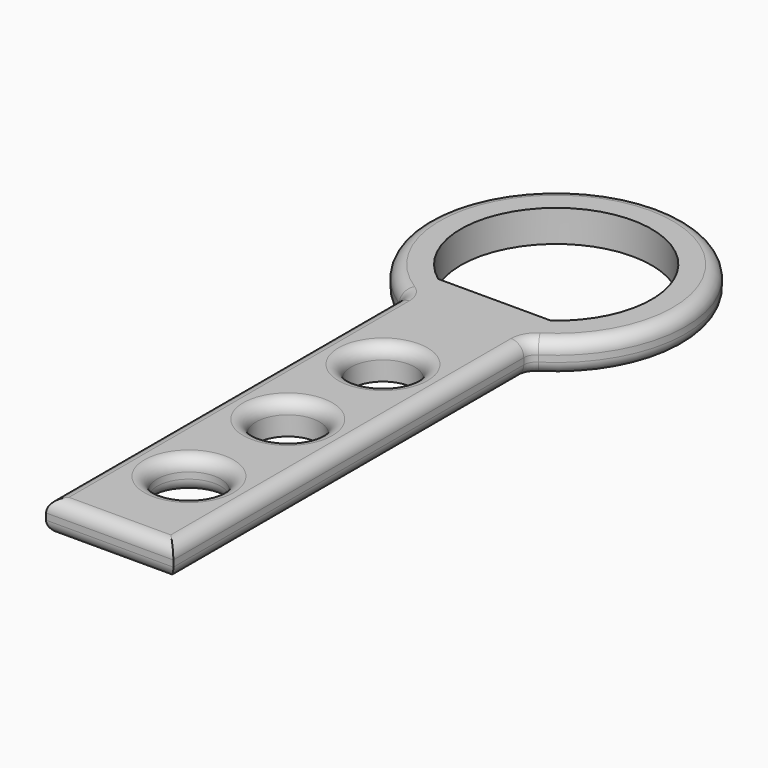
from build123d import *

# Parameters (mm, degrees)
F1_DEPTH = 5
F2_R     = 2
F3_R     = 15
F4_DEPTH = 25.4
F5_R     = 5
F6_DEPTH = 25.4
F7_R     = 2
F9_DEPTH = 5
F10_SIZE = 4.99999


# Not quite as in the source:
# - a fillet or chamfer is up to 0.001 mm smaller than in the source, because OpenCascade refuses the exact size


with BuildPart() as f1:
    # F0 (on Top) → F1 (new body)
    with BuildSketch(Plane.XY):
        with BuildLine():
            Line((-10, -35), (10, -35))
            Line((10, -35), (10, 35))
            ThreePointArc((10, 35), (0, 73.0924170341), (-10, 35))
            Line((-10, 35), (-10, -35))
        make_face()
    extrude(amount=F1_DEPTH)

    # F2
    f2_edges = [f1.edges().sort_by_distance(p)[0] for p in [
        (0, 73.092417, 5),
        (10, 0, 5),
        (-10, 0, 5),
        (0, -35, 5),
        (10, 0, 0),
        (0, 73.092417, 0),
        (-10, 0, 0),
        (-10, 35, 2.5),
        (10, 35, 2.5),
        (0, -35, 0),
    ]]
    fillet(f2_edges, radius=F2_R)

    # F3 (on face) → F4 (cut)
    with BuildSketch(Plane.XY.offset(5)):
        with Locations((0, 52.7336113155)):
            Circle(F3_R)
    extrude(amount=-F4_DEPTH, mode=Mode.SUBTRACT)

    # F5 (on face) → F6 (cut)
    with BuildSketch(Plane(origin=(0, 0, 0), x_dir=(1, 0, 0), z_dir=(0, 0, -1))):
        Circle(F5_R)
        with Locations((0, -18.6964944005)):
            Circle(F5_R)
        with Locations((0, 19.4296911359)):
            Circle(F5_R)
    extrude(amount=-F6_DEPTH, mode=Mode.SUBTRACT)

    # F7
    f7_edges = [f1.edges().sort_by_distance(p)[0] for p in [
        (-5, -19.429691, 0),
        (5, -19.429691, 2.5),
        (-5, -19.429691, 5),
        (-5, 0, 5),
        (-5, 18.696494, 5),
    ]]
    fillet(f7_edges, radius=F7_R)

    # F8 (on face) → F9 (join)
    with BuildSketch(Plane(origin=(0, 0, 0), x_dir=(1, 0, 0), z_dir=(0, 0, -1))):
        with BuildLine():
            ThreePointArc((13.2130736886, -45.6332814852), (0, -37.7336113155), (-13.2130736886, -45.6332814852))
            Line((-13.2130736886, -45.6332814852), (13.2130736886, -45.6332814852))
        make_face()
    extrude(amount=-F9_DEPTH)

    # F10 (size 5 in the source; OpenCascade refuses exactly that, so slightly less here)
    f10_edges = [f1.edges().sort_by_distance(p)[0] for p in [
        (0, 45.633281, 5),
    ]]
    chamfer(f10_edges, length=F10_SIZE)


solid = f1.part
